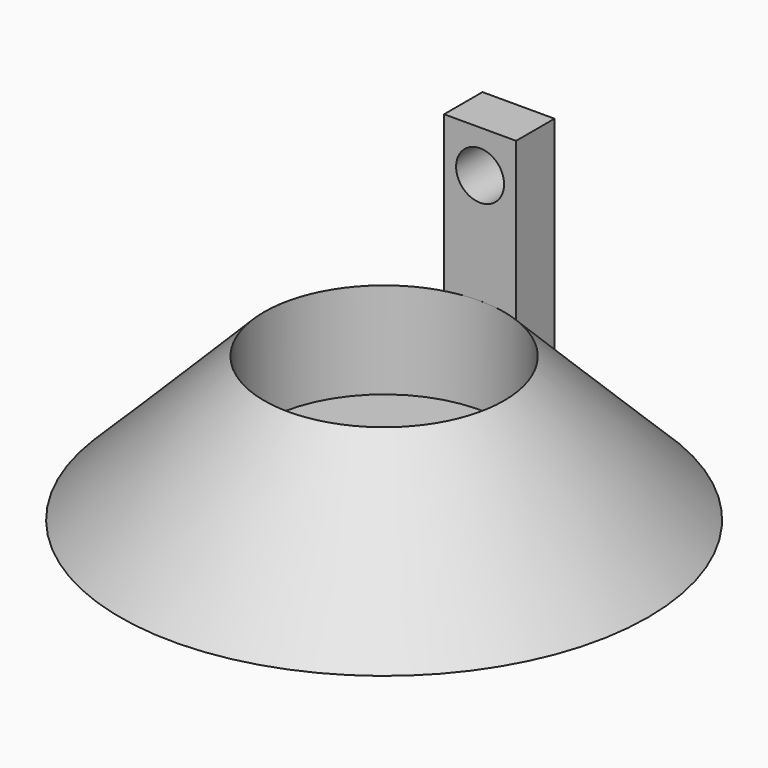
from build123d import *

# Parameters (mm, degrees)
F0_R     = 5.5
F0_R_2   = 2.5
F1_DEPTH = 3
F2_DEPTH = 1
F3_SIZE  = 2.99999
F4_W     = 1.5
F4_H     = 1
F5_DEPTH = 6.18
F6_R     = 0.5
F7_DEPTH = 25


# Not quite as in the source:
# - a fillet or chamfer is up to 0.001 mm smaller than in the source, because OpenCascade refuses the exact size


with BuildPart() as f1:
    # F0 (on Top) → F1 (new body)
    with BuildSketch(Plane.XY):
        Circle(F0_R)
        Circle(F0_R_2, mode=Mode.SUBTRACT)
    extrude(amount=F1_DEPTH)

    # F0 (on Top) → F2 (join)
    with BuildSketch(Plane.XY):
        Circle(F0_R_2)
    extrude(amount=F2_DEPTH)

    # F3 (size 3 in the source; OpenCascade refuses exactly that, so slightly less here)
    f3_edges = [f1.edges().sort_by_distance(p)[0] for p in [
        (-5.5, 0, 3),
    ]]
    chamfer(f3_edges, length=F3_SIZE)

    # F4 (on Top) → F5 (join)
    with BuildSketch(Plane.XY):
        with Locations((0, 3)):
            Rectangle(F4_W, F4_H)
    extrude(amount=F5_DEPTH)

    # F6 (on face) → F7 (cut)
    with BuildSketch(Plane.XZ.offset(-2.5)):
        with Locations((0, 5.3)):
            Circle(F6_R)
    extrude(amount=-F7_DEPTH, mode=Mode.SUBTRACT)


solid = f1.part
